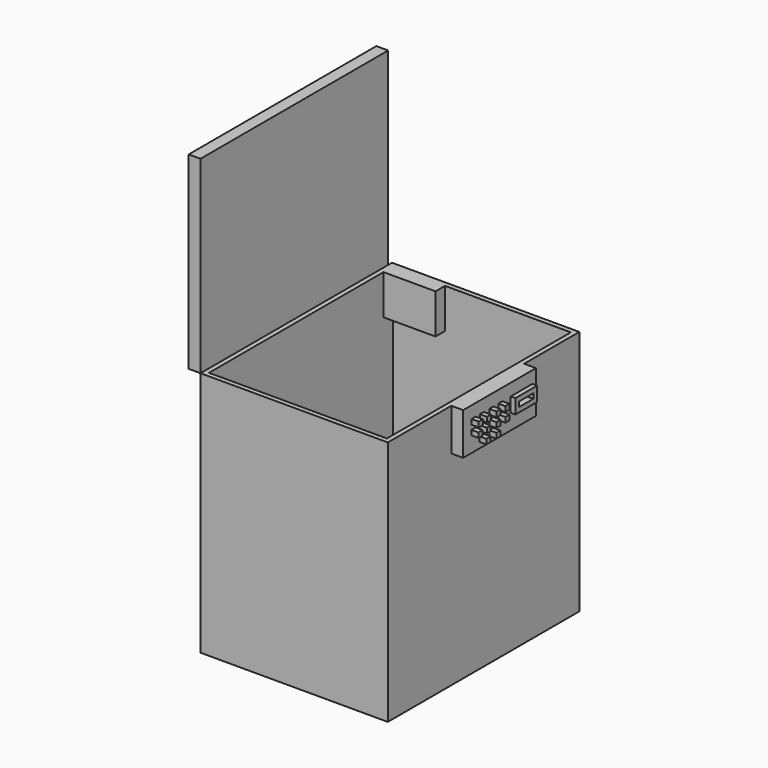
from build123d import *

# Parameters (mm, degrees)
F0_W          = 128.5288762301
F0_H          = 132.1100722998
F1_DEPTH      = 100.584
F2_T          = -2.54
F3_W          = 125.9559132159
F3_H          = 101.376414299
F4_DEPTH      = 6.35
F5_W          = 27.9540398782
F5_H          = 21.3589221239
F6_DEPTH      = 6.35
F7_W          = 48.8489195704
F7_H          = 22.5596278906
F8_DEPTH      = 6.35
F9_W          = 2.762068063
F9_H          = 2.7620643377
F9_W_2        = 2.6305429637
F9_H_2        = 2.7620717883
F9_W_3        = 2.7620717883
F9_W_4        = 2.630546689
F9_W_5        = 2.8935968876
F9_H_3        = 2.630546689
F9_H_4        = 2.6305392385
F10_DEPTH     = 3.81
F11_W         = 15.6517345458
F11_H         = 4.7349780798
F12_DEPTH     = 5.08
F13_W         = 14.5478118211
F13_H         = 7.7390819788
F14_DEPTH     = 2.54
F15_T         = 2.54
F15_T3_DEPTH  = 27.6396278906
F15_T5_DEPTH  = 53.9289195704
F15_T7_DEPTH  = 7.9735968876
F15_T9_DEPTH  = 7.710546689
F15_T11_DEPTH = 7.710546689
F15_T13_DEPTH = 7.8420717883
F15_T15_DEPTH = 7.7105429637
F15_T17_DEPTH = 7.8420717883
F15_T19_DEPTH = 7.8420717883
F15_T21_DEPTH = 7.842068063
F15_T23_DEPTH = 7.842068063
F15_T25_DEPTH = 7.7105392385
F15_T27_DEPTH = 7.842068063
F15_T29_DEPTH = 7.8420643377
F15_T31_DEPTH = 7.7105429637
F15_T33_DEPTH = 7.8420717883
F15_T35_DEPTH = 7.8420717883
F15_T37_DEPTH = 7.842068063
F15_T39_DEPTH = 19.6278118211
F15_T41_DEPTH = 12.8190819788
F15_T43_DEPTH = 134.6500722998
F15_T45_DEPTH = 100.584
F15_T47_DEPTH = 113.2911501759
F15_T49_DEPTH = 33.0340398782
F15_T51_DEPTH = 26.4389221239
F15_T53_DEPTH = 11.43
F15_T55_DEPTH = 128.5288762301


# Not quite as in the source:
# - a shell that OpenCascade refuses in one call is made with other operations: the cavity is built on its own and cut out


with BuildPart() as f1:
    # F0 (on Right) → F1 (new body)
    with BuildSketch(Plane.YZ):
        with Locations((-46.36219237, 59.4891095534)):
            Rectangle(F0_W, F0_H)
    extrude(amount=F1_DEPTH)

    # F2
    f2_openings = [f1.faces().sort_by_distance(p)[0] for p in [
        (50.292, -46.362192, 125.544146),
    ]]
    offset(amount=F2_T, openings=f2_openings)

    # F5 (on face) → F6 (join)
    with BuildSketch(Plane.XZ.offset(-15.3622457451)):
        with Locations((16.5170199391, 114.8646846414)):
            Rectangle(F5_W, F5_H)
    extrude(amount=F6_DEPTH)

    # F7 (on face) → F8 (join)
    with BuildSketch(Plane.YZ.offset(100.584)):
        with Locations((-43.5713417828, 114.264331758)):
            Rectangle(F7_W, F7_H)
    extrude(amount=F8_DEPTH)

    # F9 (on face) → F10 (join)
    with BuildSketch(Plane.YZ.offset(106.934)):
        with Locations((-60.9435793012, 117.6858767867)):
            Rectangle(F9_W, F9_H)
        with Locations((-55.4852019995, 117.6858730614)):
            Rectangle(F9_W_2, F9_H_2)
        with Locations((-49.1061359644, 117.6858730614)):
            Rectangle(F9_W_3, F9_H_2)
        with Locations((-43.0558864027, 117.6858730614)):
            Rectangle(F9_W, F9_H_2)
        with Locations((-43.0394452997, 112.6056425273)):
            Rectangle(F9_W, F9_H_2)
        with Locations((-49.0896948613, 112.6056425273)):
            Rectangle(F9_W_3, F9_H_2)
        with Locations((-49.171898514, 107.5582839549)):
            Rectangle(F9_W_4, F9_H_2)
        with Locations((-55.748257786, 107.4925214052)):
            Rectangle(F9_W_5, F9_H_3)
        with Locations((-55.600289721, 112.6056425273)):
            Rectangle(F9_W_2, F9_H_2)
        with Locations((-61.0586670227, 112.6714088023)):
            Rectangle(F9_W, F9_H_4)
    extrude(amount=F10_DEPTH)

    # F11 (on face) → F12 (join)
    with BuildSketch(Plane.YZ.offset(106.934)):
        with Locations((-28.7194242701, 116.8309524655)):
            Rectangle(F11_W, F11_H)
    extrude(amount=-F12_DEPTH)

    # F13 (on face) → F14 (join)
    with BuildSketch(Plane.YZ.offset(106.934)):
        with Locations((-28.8104629144, 115.1973679662)):
            Rectangle(F13_W, F13_H)
    extrude(amount=F14_DEPTH)

    # F15: shell of thickness 2.54, made by hand


with BuildPart() as f4:
    # F3 (on face) → F4 (new body)
    with BuildSketch(Plane(origin=(0, 0, 0), x_dir=(0, -1, 0), z_dir=(-1, 0, 0))):
        with Locations((47.6486738771, 176.2323528528)):
            Rectangle(F3_W, F3_H)
    extrude(amount=F4_DEPTH)


with BuildPart() as f15_core1:
    # F15_t2: copy of F1
    add(f1.part)

    # the walls: a layer under each face that stays
    f15_faces = [f15_core1.faces().sort_by_distance(p)[0] for p in [
        (50.292, -110.6266304851, 59.4891095534),
        (99.2958571429, 8.7216117286, 125.5441457033),
        (50.292, -46.36219237, -6.5659265965),
        (0, -46.36219237, 59.4891095534),
        (100.584, -46.36219237, 59.4891095534),
        (50.292, 17.9022457451, 59.4891095534),
        (103.759, -19.1468819976, 114.264331758),
        (106.934, -43.5713417828, 114.264331758),
        (103.759, -67.995801568, 114.264331758),
        (50.292, 15.3622457451, 60.7591095534),
        (30.4940398782, 12.1872457451, 114.8646846414),
        (16.5170199391, 9.0122457451, 114.8646846414),
        (2.54, -46.36219237, 60.7591095534),
        (50.292, -108.0866304851, 60.7591095534),
        (98.044, -46.36219237, 60.7591095534),
        (103.759, -43.5713417828, 102.9845178127),
        (108.839, -55.748257786, 108.8077947497),
        (108.839, -54.3014593422, 107.4925214052),
        (108.839, -57.1950562298, 107.4925214052),
        (108.839, -55.748257786, 106.1772480607),
        (108.839, -49.171898514, 108.939319849),
        (108.839, -47.8566251695, 107.5582839549),
        (108.839, -50.4871718585, 107.5582839549),
        (108.839, -49.171898514, 106.1772480607),
        (108.839, -55.600289721, 113.9866784215),
        (108.839, -54.2850182392, 112.6056425273),
        (108.839, -56.9155612029, 112.6056425273),
        (108.839, -55.600289721, 111.2246066332),
        (108.839, -49.0896948613, 113.9866784215),
        (108.839, -47.7086589672, 112.6056425273),
        (108.839, -50.4707307555, 112.6056425273),
        (108.839, -49.0896948613, 111.2246066332),
        (108.839, -43.0394452997, 113.9866784215),
        (108.839, -41.6584112681, 112.6056425273),
        (108.839, -44.4204793312, 112.6056425273),
        (108.839, -43.0394452997, 111.2246066332),
        (108.839, -61.0586670227, 111.356139183),
        (108.839, -62.4397010542, 112.6714088023),
        (108.839, -59.6776329912, 112.6714088023),
        (108.839, -61.0586670227, 113.9866784215),
        (108.839, -60.9435793012, 119.0669089556),
        (108.839, -59.5625452697, 117.6858767867),
        (108.839, -62.3246133327, 117.6858767867),
        (108.839, -60.9435793012, 116.3048446178),
        (108.839, -55.4852019995, 119.0669089556),
        (108.839, -54.1699305177, 117.6858730614),
        (108.839, -56.8004734814, 117.6858730614),
        (108.839, -55.4852019995, 116.3048371673),
        (108.839, -49.1061359644, 119.0669089556),
        (108.839, -47.7251000702, 117.6858730614),
        (108.839, -50.4871718585, 117.6858730614),
        (108.839, -49.1061359644, 116.3048371673),
        (108.839, -43.0558864027, 119.0669089556),
        (108.839, -41.6748523712, 117.6858730614),
        (108.839, -44.4369204342, 117.6858730614),
        (108.839, -43.0558864027, 116.3048371673),
        (108.204, -28.8104629144, 119.0669089556),
        (108.204, -36.084368825, 115.1973679662),
        (108.204, -28.8104629144, 111.3278269768),
        (108.204, -21.5365570039, 115.1973679662),
        (50.292, -46.36219237, -4.0259265965),
        (16.5170199391, 12.1872457451, 104.1852235794),
        (110.744, -55.748257786, 107.4925214052),
        (110.744, -49.171898514, 107.5582839549),
        (110.744, -55.600289721, 112.6056425273),
        (110.744, -49.0896948613, 112.6056425273),
        (110.744, -43.0394452997, 112.6056425273),
        (110.744, -61.0586670227, 112.6714088023),
        (110.744, -60.9435793012, 117.6858767867),
        (110.744, -55.4852019995, 117.6858730614),
        (110.744, -49.1061359644, 117.6858730614),
        (110.744, -43.0558864027, 117.6858730614),
    ]]
    thicken(f15_faces, amount=-F15_T, mode=Mode.SUBTRACT)

    # F15_s4 → F15_t3 (cut)
    with BuildSketch(Plane.XY.offset(100.4445178127)):
        Polygon((100.6094, -68.021201568), (98.044, -67.995801568), (98.044, -65.455801568), (100.584, -65.455801568), align=None)
        Polygon((100.6094, -19.1214819976), (98.044, -19.1468819976), (98.044, -21.6868819976), (100.584, -21.6868819976), align=None)
    extrude(amount=F15_T3_DEPTH, mode=Mode.SUBTRACT)

    # F15_s6 → F15_t5 (cut)
    with BuildSketch(Plane.XZ.offset(16.6068819976)):
        Polygon((100.6094, 102.9591178127), (98.044, 102.9845178127), (98.044, 105.5245178127), (100.584, 105.5245178127), align=None)
    extrude(amount=F15_T5_DEPTH, mode=Mode.SUBTRACT)

    # F15_s8 → F15_t7 (cut)
    with BuildSketch(Plane.XZ.offset(51.7614593422)):
        Polygon((106.9594, 108.8331947497), (104.394, 108.8077947497), (104.394, 106.2677947497), (106.934, 106.2677947497), align=None)
        Polygon((106.9594, 106.1518480607), (104.394, 106.1772480607), (104.394, 108.7172480607), (106.934, 108.7172480607), align=None)
    extrude(amount=F15_T7_DEPTH, mode=Mode.SUBTRACT)

    # F15_s10 → F15_t9 (cut)
    with BuildSketch(Plane.XY.offset(103.6372480607)):
        Polygon((106.9594, -54.2760593422), (104.394, -54.3014593422), (104.394, -56.8414593422), (106.934, -56.8414593422), align=None)
        Polygon((106.9594, -57.2204562298), (104.394, -57.1950562298), (104.394, -54.6550562298), (106.934, -54.6550562298), align=None)
    extrude(amount=F15_T9_DEPTH, mode=Mode.SUBTRACT)

    # F15_s12 → F15_t11 (cut)
    with BuildSketch(Plane.XZ.offset(45.3166251695)):
        Polygon((106.9594, 108.964719849), (104.394, 108.939319849), (104.394, 106.399319849), (106.934, 106.399319849), align=None)
        Polygon((106.9594, 106.1518480607), (104.394, 106.1772480607), (104.394, 108.7172480607), (106.934, 108.7172480607), align=None)
    extrude(amount=F15_T11_DEPTH, mode=Mode.SUBTRACT)

    # F15_s14 → F15_t13 (cut)
    with BuildSketch(Plane.XY.offset(103.6372480607)):
        Polygon((106.9594, -47.8312251695), (104.394, -47.8566251695), (104.394, -50.3966251695), (106.934, -50.3966251695), align=None)
        Polygon((106.9594, -50.5125718585), (104.394, -50.4871718585), (104.394, -47.9471718585), (106.934, -47.9471718585), align=None)
    extrude(amount=F15_T13_DEPTH, mode=Mode.SUBTRACT)

    # F15_s16 → F15_t15 (cut)
    with BuildSketch(Plane.XZ.offset(51.7450182392)):
        Polygon((106.9594, 114.0120784215), (104.394, 113.9866784215), (104.394, 111.4466784215), (106.934, 111.4466784215), align=None)
        Polygon((106.9594, 111.1992066332), (104.394, 111.2246066332), (104.394, 113.7646066332), (106.934, 113.7646066332), align=None)
    extrude(amount=F15_T15_DEPTH, mode=Mode.SUBTRACT)

    # F15_s18 → F15_t17 (cut)
    with BuildSketch(Plane.XY.offset(108.6846066332)):
        Polygon((106.9594, -54.2596182392), (104.394, -54.2850182392), (104.394, -56.8250182392), (106.934, -56.8250182392), align=None)
        Polygon((106.9594, -56.9409612029), (104.394, -56.9155612029), (104.394, -54.3755612029), (106.934, -54.3755612029), align=None)
        Polygon((106.9594, -47.6832589672), (104.394, -47.7086589672), (104.394, -50.2486589672), (106.934, -50.2486589672), align=None)
        Polygon((106.9594, -50.4961307555), (104.394, -50.4707307555), (104.394, -47.9307307555), (106.934, -47.9307307555), align=None)
        Polygon((106.9594, -41.6330112681), (104.394, -41.6584112681), (104.394, -44.1984112681), (106.934, -44.1984112681), align=None)
        Polygon((106.9594, -44.4458793312), (104.394, -44.4204793312), (104.394, -41.8804793312), (106.934, -41.8804793312), align=None)
    extrude(amount=F15_T17_DEPTH, mode=Mode.SUBTRACT)

    # F15_s20 → F15_t19 (cut)
    with BuildSketch(Plane.XZ.offset(45.1686589672)):
        Polygon((106.9594, 114.0120784215), (104.394, 113.9866784215), (104.394, 111.4466784215), (106.934, 111.4466784215), align=None)
        Polygon((106.9594, 111.1992066332), (104.394, 111.2246066332), (104.394, 113.7646066332), (106.934, 113.7646066332), align=None)
    extrude(amount=F15_T19_DEPTH, mode=Mode.SUBTRACT)

    # F15_s22 → F15_t21 (cut)
    with BuildSketch(Plane.XZ.offset(39.1184112681)):
        Polygon((106.9594, 114.0120784215), (104.394, 113.9866784215), (104.394, 111.4466784215), (106.934, 111.4466784215), align=None)
        Polygon((106.9594, 111.1992066332), (104.394, 111.2246066332), (104.394, 113.7646066332), (106.934, 113.7646066332), align=None)
    extrude(amount=F15_T21_DEPTH, mode=Mode.SUBTRACT)

    # F15_s24 → F15_t23 (cut)
    with BuildSketch(Plane.XZ.offset(57.1376329912)):
        Polygon((106.9594, 111.330739183), (104.394, 111.356139183), (104.394, 113.896139183), (106.934, 113.896139183), align=None)
        Polygon((106.9594, 114.0120784215), (104.394, 113.9866784215), (104.394, 111.4466784215), (106.934, 111.4466784215), align=None)
    extrude(amount=F15_T23_DEPTH, mode=Mode.SUBTRACT)

    # F15_s26 → F15_t25 (cut)
    with BuildSketch(Plane.XY.offset(108.816139183)):
        Polygon((106.9594, -62.4651010542), (104.394, -62.4397010542), (104.394, -59.8997010542), (106.934, -59.8997010542), align=None)
        Polygon((106.9594, -59.6522329912), (104.394, -59.6776329912), (104.394, -62.2176329912), (106.934, -62.2176329912), align=None)
    extrude(amount=F15_T25_DEPTH, mode=Mode.SUBTRACT)

    # F15_s28 → F15_t27 (cut)
    with BuildSketch(Plane.XZ.offset(57.0225452697)):
        Polygon((106.9594, 119.0923089556), (104.394, 119.0669089556), (104.394, 116.5269089556), (106.934, 116.5269089556), align=None)
        Polygon((106.9594, 116.2794446178), (104.394, 116.3048446178), (104.394, 118.8448446178), (106.934, 118.8448446178), align=None)
    extrude(amount=F15_T27_DEPTH, mode=Mode.SUBTRACT)

    # F15_s30 → F15_t29 (cut)
    with BuildSketch(Plane.XY.offset(113.7648446178)):
        Polygon((106.9594, -59.5371452697), (104.394, -59.5625452697), (104.394, -62.1025452697), (106.934, -62.1025452697), align=None)
        Polygon((106.9594, -62.3500133327), (104.394, -62.3246133327), (104.394, -59.7846133327), (106.934, -59.7846133327), align=None)
    extrude(amount=F15_T29_DEPTH, mode=Mode.SUBTRACT)

    # F15_s32 → F15_t31 (cut)
    with BuildSketch(Plane.XZ.offset(51.6299305177)):
        Polygon((106.9594, 119.0923089556), (104.394, 119.0669089556), (104.394, 116.5269089556), (106.934, 116.5269089556), align=None)
        Polygon((106.9594, 116.2794371673), (104.394, 116.3048371673), (104.394, 118.8448371673), (106.934, 118.8448371673), align=None)
    extrude(amount=F15_T31_DEPTH, mode=Mode.SUBTRACT)

    # F15_s34 → F15_t33 (cut)
    with BuildSketch(Plane.XY.offset(113.7648371673)):
        Polygon((106.9594, -54.1445305177), (104.394, -54.1699305177), (104.394, -56.7099305177), (106.934, -56.7099305177), align=None)
        Polygon((106.9594, -56.8258734814), (104.394, -56.8004734814), (104.394, -54.2604734814), (106.934, -54.2604734814), align=None)
        Polygon((106.9594, -47.6997000702), (104.394, -47.7251000702), (104.394, -50.2651000702), (106.934, -50.2651000702), align=None)
        Polygon((106.9594, -50.5125718585), (104.394, -50.4871718585), (104.394, -47.9471718585), (106.934, -47.9471718585), align=None)
        Polygon((106.9594, -41.6494523712), (104.394, -41.6748523712), (104.394, -44.2148523712), (106.934, -44.2148523712), align=None)
        Polygon((106.9594, -44.4623204342), (104.394, -44.4369204342), (104.394, -41.8969204342), (106.934, -41.8969204342), align=None)
    extrude(amount=F15_T33_DEPTH, mode=Mode.SUBTRACT)

    # F15_s36 → F15_t35 (cut)
    with BuildSketch(Plane.XZ.offset(45.1851000702)):
        Polygon((106.9594, 119.0923089556), (104.394, 119.0669089556), (104.394, 116.5269089556), (106.934, 116.5269089556), align=None)
        Polygon((106.9594, 116.2794371673), (104.394, 116.3048371673), (104.394, 118.8448371673), (106.934, 118.8448371673), align=None)
    extrude(amount=F15_T35_DEPTH, mode=Mode.SUBTRACT)

    # F15_s38 → F15_t37 (cut)
    with BuildSketch(Plane.XZ.offset(39.1348523712)):
        Polygon((106.9594, 119.0923089556), (104.394, 119.0669089556), (104.394, 116.5269089556), (106.934, 116.5269089556), align=None)
        Polygon((106.9594, 116.2794371673), (104.394, 116.3048371673), (104.394, 118.8448371673), (106.934, 118.8448371673), align=None)
    extrude(amount=F15_T37_DEPTH, mode=Mode.SUBTRACT)

    # F15_s40 → F15_t39 (cut)
    with BuildSketch(Plane.XZ.offset(18.9965570039)):
        Polygon((106.9594, 119.0923089556), (104.394, 119.0669089556), (104.394, 116.5269089556), (106.934, 116.5269089556), align=None)
        Polygon((106.9594, 111.3024269768), (104.394, 111.3278269768), (104.394, 113.8678269768), (106.934, 113.8678269768), align=None)
    extrude(amount=F15_T39_DEPTH, mode=Mode.SUBTRACT)

    # F15_s42 → F15_t41 (cut)
    with BuildSketch(Plane.XY.offset(108.7878269768)):
        Polygon((106.9594, -36.109768825), (104.394, -36.084368825), (104.394, -33.544368825), (106.934, -33.544368825), align=None)
        Polygon((106.9594, -21.5111570039), (104.394, -21.5365570039), (104.394, -24.0765570039), (106.934, -24.0765570039), align=None)
    extrude(amount=F15_T41_DEPTH, mode=Mode.SUBTRACT)

    # F15_s44 → F15_t43 (cut)
    with BuildSketch(Plane.XY.offset(-6.5659265965)):
        Polygon((98.0186, 15.3368457451), (98.044, 17.9022457451), (100.584, 17.9022457451), (100.584, 15.3622457451), align=None)
        Polygon((2.5654, -108.0612304851), (0, -108.0866304851), (0, -110.6266304851), (2.54, -110.6266304851), align=None)
        Polygon((98.0186, -108.0612304851), (98.044, -110.6266304851), (100.584, -110.6266304851), (100.584, -108.0866304851), align=None)
    extrude(amount=F15_T43_DEPTH, mode=Mode.SUBTRACT)

    # F15_s46 → F15_t45 (cut)
    with BuildSketch(Plane.YZ):
        Polygon((15.3368457451, -4.0005265965), (17.9022457451, -4.0259265965), (17.9022457451, -6.5659265965), (15.3622457451, -6.5659265965), align=None)
        Polygon((-108.0612304851, -4.0005265965), (-110.6266304851, -4.0259265965), (-110.6266304851, -6.5659265965), (-108.0866304851, -6.5659265965), align=None)
    extrude(amount=F15_T45_DEPTH, mode=Mode.SUBTRACT)

    # F15_s48 → F15_t47 (cut)
    with BuildSketch(Plane.XY.offset(-6.5659265965)):
        Polygon((2.5654, 15.3368457451), (2.54, 17.9022457451), (0, 17.9022457451), (0, 15.3622457451), align=None)
    extrude(amount=F15_T47_DEPTH, mode=Mode.SUBTRACT)

    # F15_s50 → F15_t49 (cut)
    with BuildSketch(Plane.YZ):
        Polygon((15.3368457451, 104.1598235794), (17.9022457451, 104.1852235794), (17.9022457451, 106.7252235794), (15.3622457451, 106.7252235794), align=None)
    extrude(amount=F15_T49_DEPTH, mode=Mode.SUBTRACT)

    # F15_s52 → F15_t51 (cut)
    with BuildSketch(Plane.XY.offset(101.6452235794)):
        Polygon((30.5194398782, 15.3368457451), (30.4940398782, 17.9022457451), (27.9540398782, 17.9022457451), (27.9540398782, 15.3622457451), align=None)
        Polygon((2.5654, 8.9868457451), (2.54, 11.5522457451), (0, 11.5522457451), (0, 9.0122457451), align=None)
    extrude(amount=F15_T51_DEPTH, mode=Mode.SUBTRACT)

    # F15_s54 → F15_t53 (cut)
    with BuildSketch(Plane.XZ.offset(-17.9022457451)):
        Polygon((2.5654, 104.1598235794), (0, 104.1852235794), (0, 106.7252235794), (2.54, 106.7252235794), align=None)
    extrude(amount=F15_T53_DEPTH, mode=Mode.SUBTRACT)

    # F15_s56 → F15_t55 (cut)
    with BuildSketch(Plane.XZ.offset(-17.9022457451)):
        Polygon((2.5654, -4.0005265965), (0, -4.0259265965), (0, -6.5659265965), (2.54, -6.5659265965), align=None)
        Polygon((98.0186, -4.0005265965), (100.584, -4.0259265965), (100.584, -6.5659265965), (98.044, -6.5659265965), align=None)
    extrude(amount=F15_T55_DEPTH, mode=Mode.SUBTRACT)


with BuildPart() as f1_1:
    add(f1.part)

    # what is left inside the walls is the cavity
    f15_cavity = [f15_core1.part.solids().sort_by_distance(p)[0] for p in [
        (15.24702, 11.577646, 112.151531),
        (100.6094, -43.571342, 111.35106),
    ]]
    add(f15_cavity, mode=Mode.SUBTRACT)


solid = Compound([f4.part, f1_1.part])
